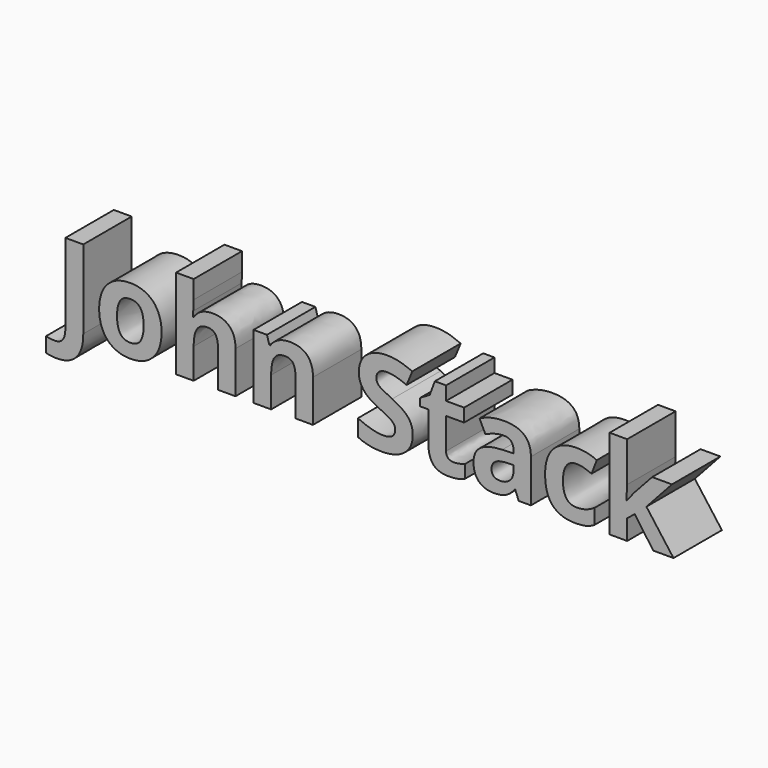
from build123d import *

# Parameters (mm, degrees)
F0_TEXT_SIZE = 19.4918194444
F1_DEPTH     = 10


# Not quite as in the source:
# - Text() gives the source's letters only with a copy of the font that has no kerning and outlines rounded to 1/6400 em; it was checked with that copy


with BuildPart() as f1:
    # F0 (on Front) → F1 (new body)
    with BuildSketch(Plane.XZ):
        with Locations((4.0000051302, 14.482945)):
            Text('John Stack', F0_TEXT_SIZE, font='Open Sans', font_style=FontStyle.BOLD, text_align=(TextAlign.LEFT, TextAlign.BOTTOM))
    extrude(amount=F1_DEPTH)


solid = f1.part
